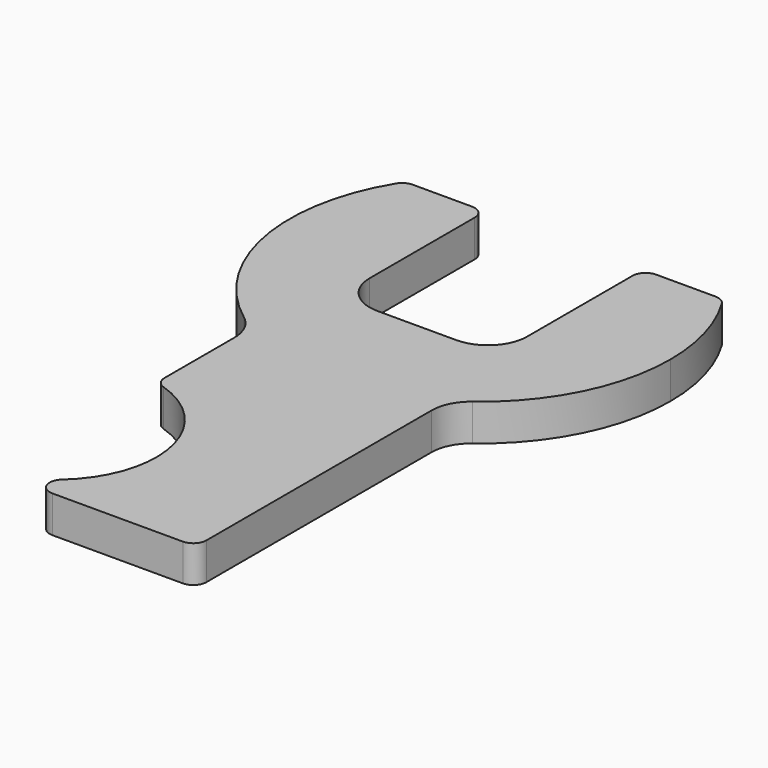
from build123d import *

# Parameters (mm, degrees)
F1_DEPTH = 2.8
F2_R     = 3
F3_R     = 1


with BuildPart() as f1:
    # F0 (on Top) → F1 (new body)
    with BuildSketch(Plane.XY):
        with BuildLine():
            ThreePointArc((7.5, -12.3924725737), (12.6186961846, -7.1127971356), (14.4852813742, 0))
            ThreePointArc((14.4852813742, 0), (13.869819685, 4.1774966664), (12.075735029, 8))
            Line((12.075735029, 8), (6, 8))
            Line((6, 8), (6, 6))
            Line((6, 6), (6, -6))
            Line((6, -6), (-6, -6))
            Line((-6, -6), (-6, 6))
            Line((-6, 6), (-6, 8))
            Line((-6, 8), (-12.075735029, 8))
            ThreePointArc((-12.075735029, 8), (-14.1338453684, -3.1714021492), (-7.5, -12.3924725737))
            Line((-7.5, -12.3924725737), (7.5, -12.3924725737))
        make_face()
        with BuildLine():
            Line((7.5, -36.3924725737), (7.5, -12.3924725737))
            ThreePointArc((7.5, -12.3924725737), (0, -14.4852813742), (-7.5, -12.3924725737))
            Line((-7.5, -12.3924725737), (-7.5, -21.3924725737))
            ThreePointArc((-7.5, -21.3924725737), (-1.5, -28.8924725737), (-7.5, -36.3924725737))
            Line((-7.5, -36.3924725737), (7.5, -36.3924725737))
        make_face()
        with BuildLine():
            ThreePointArc((-7.5, -12.3924725737), (0, -14.4852813742), (7.5, -12.3924725737))
            Line((7.5, -12.3924725737), (-7.5, -12.3924725737))
        make_face()
    extrude(amount=F1_DEPTH)

    # F2
    f2_edges = [f1.edges().sort_by_distance(p)[0] for p in [
        (-7.5, -12.392473, 1.4),
        (7.5, -12.392473, 1.4),
        (6, -6, 1.4),
        (-6, -6, 1.4),
    ]]
    fillet(f2_edges, radius=F2_R)

    # F3
    f3_edges = [f1.edges().sort_by_distance(p)[0] for p in [
        (-7.5, -36.392473, 1.4),
        (7.5, -36.392473, 1.4),
        (6, 8, 1.4),
        (-6, 8, 1.4),
        (-12.075735, 8, 1.4),
        (12.075735, 8, 1.4),
        (-7.5, -21.392473, 1.4),
    ]]
    fillet(f3_edges, radius=F3_R)


solid = f1.part
